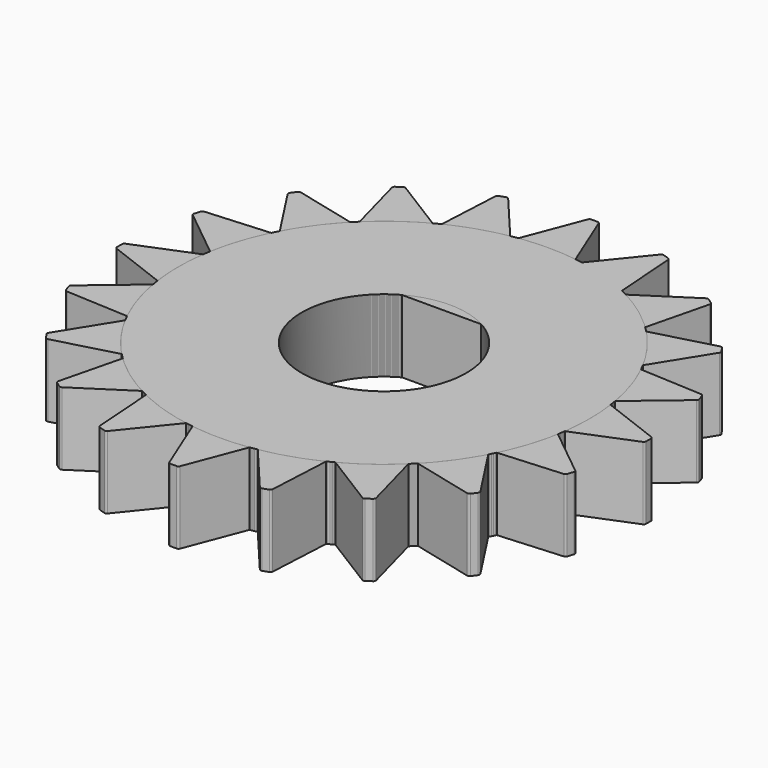
from build123d import *

# Parameters (mm, degrees)
F1_DEPTH = 3
F3_COUNT = 20
F4_DEPTH = 3


# Not quite as in the source:
# - a feature names something its author has since deleted; it is built from what else it names


with BuildPart() as f1:
    # F0 (on Top) → F1 (new body)
    with BuildSketch(Plane.XY):
        with BuildLine():
            ThreePointArc((-1.1790691115, 8.417826087), (-5.5779885511, -6.4137386698), (8.5, 0))
            ThreePointArc((8.5, 0), (6.4137386698, 5.5779885511), (1.1790691115, 8.417826087))
            ThreePointArc((1.1790691115, 8.417826087), (0, 8.5), (-1.1790691115, 8.417826087))
        make_face()
        with BuildLine():
            ThreePointArc((1.65, 2.9727932992), (2.9300170648, 1.7248188311), (3.4, 0))
            ThreePointArc((3.4, 0), (-1.7248188311, -2.9300170648), (-1.65, 2.9727932992))
            ThreePointArc((-1.65, 2.9727932992), (0, 3.4), (1.65, 2.9727932992))
        make_face(mode=Mode.SUBTRACT)
        with BuildLine():
            ThreePointArc((-1.1790691115, 8.417826087), (0, 8.5), (1.1790691115, 8.417826087))
            Line((1.1790691115, 8.417826087), (0.1921873111, 10.8473598172))
            ThreePointArc((0.1921873111, 10.8473598172), (0.1553808933, 10.8926819004), (0.0995391073, 10.9097259185))
            Line((0.0995391073, 10.9097259185), (-0.156993363, 10.9097259185))
            ThreePointArc((-0.156993363, 10.9097259185), (-0.2136813833, 10.8921059425), (-0.2503925725, 10.8454552856))
            Line((-0.2503925725, 10.8454552856), (-1.1790691115, 8.417826087))
        make_face()
    extrude(amount=F1_DEPTH)


with BuildPart() as f3_1:
    # F3: instance of F1
    add(f1.part.rotate(Axis((0, 0, 10.8799347654), (0, 0, 1)), 1 * 360 / F3_COUNT))


with BuildPart() as f3_2:
    # F3: instance of F1
    add(f1.part.rotate(Axis((0, 0, 10.8799347654), (0, 0, 1)), 2 * 360 / F3_COUNT))


with BuildPart() as f3_3:
    # F3: instance of F1
    add(f1.part.rotate(Axis((0, 0, 10.8799347654), (0, 0, 1)), 3 * 360 / F3_COUNT))


with BuildPart() as f3_4:
    # F3: instance of F1
    add(f1.part.rotate(Axis((0, 0, 10.8799347654), (0, 0, 1)), 4 * 360 / F3_COUNT))


with BuildPart() as f3_5:
    # F3: instance of F1
    add(f1.part.rotate(Axis((0, 0, 10.8799347654), (0, 0, 1)), 5 * 360 / F3_COUNT))


with BuildPart() as f3_6:
    # F3: instance of F1
    add(f1.part.rotate(Axis((0, 0, 10.8799347654), (0, 0, 1)), 6 * 360 / F3_COUNT))


with BuildPart() as f3_7:
    # F3: instance of F1
    add(f1.part.rotate(Axis((0, 0, 10.8799347654), (0, 0, 1)), 7 * 360 / F3_COUNT))


with BuildPart() as f3_8:
    # F3: instance of F1
    add(f1.part.rotate(Axis((0, 0, 10.8799347654), (0, 0, 1)), 8 * 360 / F3_COUNT))


with BuildPart() as f3_9:
    # F3: instance of F1
    add(f1.part.rotate(Axis((0, 0, 10.8799347654), (0, 0, 1)), 9 * 360 / F3_COUNT))


with BuildPart() as f3_10:
    # F3: instance of F1
    add(f1.part.rotate(Axis((0, 0, 10.8799347654), (0, 0, 1)), 10 * 360 / F3_COUNT))


with BuildPart() as f3_11:
    # F3: instance of F1
    add(f1.part.rotate(Axis((0, 0, 10.8799347654), (0, 0, 1)), 11 * 360 / F3_COUNT))


with BuildPart() as f3_12:
    # F3: instance of F1
    add(f1.part.rotate(Axis((0, 0, 10.8799347654), (0, 0, 1)), 12 * 360 / F3_COUNT))


with BuildPart() as f3_13:
    # F3: instance of F1
    add(f1.part.rotate(Axis((0, 0, 10.8799347654), (0, 0, 1)), 13 * 360 / F3_COUNT))


with BuildPart() as f3_14:
    # F3: instance of F1
    add(f1.part.rotate(Axis((0, 0, 10.8799347654), (0, 0, 1)), 14 * 360 / F3_COUNT))


with BuildPart() as f3_15:
    # F3: instance of F1
    add(f1.part.rotate(Axis((0, 0, 10.8799347654), (0, 0, 1)), 15 * 360 / F3_COUNT))


with BuildPart() as f3_16:
    # F3: instance of F1
    add(f1.part.rotate(Axis((0, 0, 10.8799347654), (0, 0, 1)), 16 * 360 / F3_COUNT))


with BuildPart() as f3_17:
    # F3: instance of F1
    add(f1.part.rotate(Axis((0, 0, 10.8799347654), (0, 0, 1)), 17 * 360 / F3_COUNT))


with BuildPart() as f3_18:
    # F3: instance of F1
    add(f1.part.rotate(Axis((0, 0, 10.8799347654), (0, 0, 1)), 18 * 360 / F3_COUNT))


with BuildPart() as f3_19:
    # F3: instance of F1
    add(f1.part.rotate(Axis((0, 0, 10.8799347654), (0, 0, 1)), 19 * 360 / F3_COUNT))


with BuildPart() as f4:
    # F0 (on Top) → F4 (new body)
    with BuildSketch(Plane.XY):
        with BuildLine():
            Line((-1.65, 2.9727932992), (1.65, 2.9727932992))
            ThreePointArc((1.65, 2.9727932992), (0, 3.4), (-1.65, 2.9727932992))
        make_face()
    extrude(amount=F4_DEPTH)


solid = Compound([f1.part, f3_1.part, f3_2.part, f3_3.part, f3_4.part, f3_5.part, f3_6.part, f3_7.part, f3_8.part, f3_9.part, f3_10.part, f3_11.part, f3_12.part, f3_13.part, f3_14.part, f3_15.part, f3_16.part, f3_17.part, f3_18.part, f3_19.part, f4.part])
